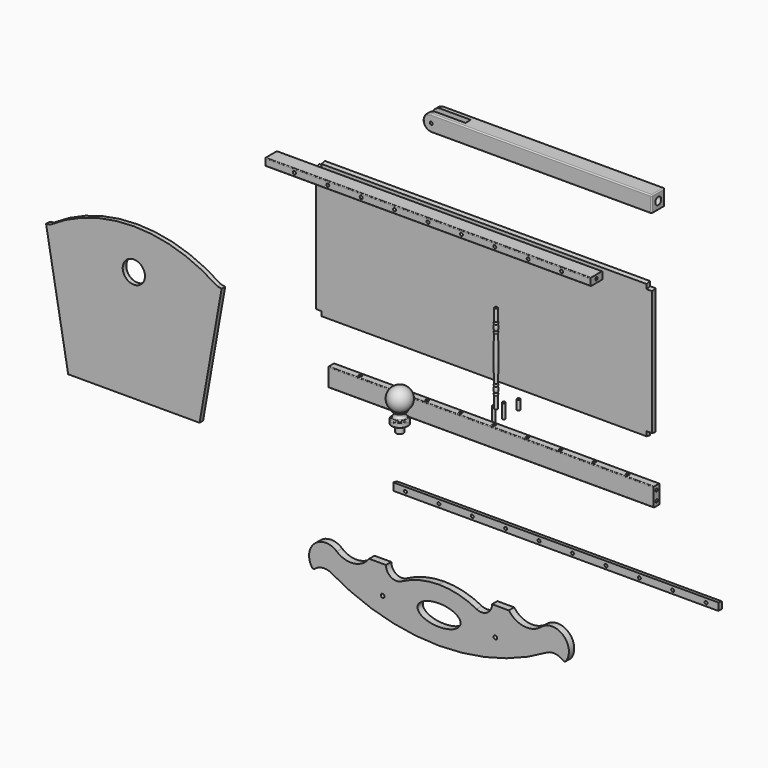
from build123d import *

# Parameters (mm, degrees)
F0_W      = 876
F0_H      = 20
F1_DEPTH  = 50
F2_R      = 4
F4_DEPTH  = 20
F5_R      = 4
F6_DEPTH  = 20
F12_DEPTH = 18
F13_R     = 5
F14_R     = 5
F15_DEPTH = 18
F16_R     = 30
F17_DEPTH = 12
F18_W     = 876
F18_H     = 20
F19_DEPTH = 40
F20_R     = 4
F21_DEPTH = 20
F22_R     = 4
F23_DEPTH = 20
F24_R     = 4
F25_DEPTH = 20
F26_R     = 2
F27_R     = 2
F28_R     = 4
F29_DEPTH = 16
F30_R     = 2
F31_R     = 4
F32_DEPTH = 39
F33_SIZE  = 0.5
F34_R     = 4
F35_DEPTH = 44
F37_DEPTH = 44
F40_DEPTH = 18
F41_R     = 4
F42_DEPTH = 180.001
F43_DEPTH = 20
F44_W     = 345
F44_H     = 12
F45_DEPTH = 12
F46_R     = 10
F47_DEPTH = 20
F48_R     = 3
F50_DEPTH = 876
F51_R     = 4
F52_DEPTH = 12
F53_R     = 4
F54_DEPTH = 27
F55_SIZE  = 1
F57_DEPTH = 906
F59_DEPTH = 15
F61_DEPTH = 15


# Not quite as in the source:
# - a pattern or mirror of a feature is missing from the dataset's text; its kind, count and spacing are read off the source's solid


with BuildPart() as f1:
    # F0 (on Top) → F1 (new body)
    with BuildSketch(Plane.XY):
        with Locations((62, 90)):
            Rectangle(F0_W, F0_H)
    extrude(amount=F1_DEPTH)

    # F2 (on face) → F4 (cut)
    with BuildSketch(Plane(origin=(-376, 0, 0), x_dir=(0, -1, 0), z_dir=(-1, 0, 0))):
        with Locations((-90, 38)):
            Circle(F2_R)
        with Locations((-90, 12)):
            Circle(F2_R)
    f4 = extrude(amount=-F4_DEPTH, mode=Mode.SUBTRACT)

    # F4_copies: F4 across plane
    add(f4.mirror(Plane(origin=(62, 0, 0), x_dir=(0, 0, 1), z_dir=(1, 0, 0))), mode=Mode.SUBTRACT)

    # F5 (on face) → F6 (cut)
    with BuildSketch(Plane.XY.offset(50)):
        with Locations((-298, 90)):
            Circle(F5_R)
        with Locations((-208, 90)):
            Circle(F5_R)
        with Locations((-118, 90)):
            Circle(F5_R)
        with Locations((-28, 90)):
            Circle(F5_R)
        with Locations((62, 90)):
            Circle(F5_R)
        with Locations((152, 90)):
            Circle(F5_R)
        with Locations((242, 90)):
            Circle(F5_R)
        with Locations((332, 90)):
            Circle(F5_R)
        with Locations((422, 90)):
            Circle(F5_R)
    extrude(amount=-F6_DEPTH, mode=Mode.SUBTRACT)

    # F27
    f27_edges = [f1.edges().sort_by_distance(p)[0] for p in [
        (62, 80, 50),
        (62, 100, 50),
        (62, 80, 0),
        (62, 100, 0),
    ]]
    fillet(f27_edges, radius=F27_R)

    # F28 (on face) → F29 (cut)
    with BuildSketch(Plane(origin=(0, 100, 0), x_dir=(-1, 0, 0), z_dir=(0, 1, 0))):
        with Locations((-467, 12)):
            Circle(F28_R)
        with Locations((-377, 12)):
            Circle(F28_R)
        with Locations((-287, 12)):
            Circle(F28_R)
        with Locations((-197, 12)):
            Circle(F28_R)
        with Locations((-107, 12)):
            Circle(F28_R)
        with Locations((-17, 12)):
            Circle(F28_R)
        with Locations((73, 12)):
            Circle(F28_R)
        with Locations((163, 12)):
            Circle(F28_R)
        with Locations((253, 12)):
            Circle(F28_R)
        with Locations((343, 12)):
            Circle(F28_R)
    extrude(amount=-F29_DEPTH, mode=Mode.SUBTRACT)


with BuildPart() as f8:
    # F7 (on Front) → F8 (revolve)
    with BuildSketch(Plane.XZ):
        with BuildLine():
            Line((139.2944970131, 150), (139.2944970131, 390))
            Line((139.2944970131, 390), (135.2944970131, 390))
            Line((135.2944970131, 390), (135.2944970131, 370))
            Line((135.2944970131, 370), (135.2944970131, 358))
            ThreePointArc((135.2944970131, 358), (134.2717225881, 354.5), (135.2944970131, 351))
            ThreePointArc((135.2944970131, 351), (133.8349932308, 343.5), (135.2944970131, 336))
            ThreePointArc((135.2944970131, 336), (134.2717225881, 332.5), (135.2944970131, 329))
            ThreePointArc((135.2944970131, 329), (133.8432027401, 270), (135.2944970131, 211))
            ThreePointArc((135.2944970131, 211), (134.2717225881, 207.5), (135.2944970131, 204))
            ThreePointArc((135.2944970131, 204), (133.8349932308, 196.5), (135.2944970131, 189))
            ThreePointArc((135.2944970131, 189), (134.2717225881, 185.5), (135.2944970131, 182))
            Line((135.2944970131, 182), (135.2944970131, 170))
            Line((135.2944970131, 170), (135.2944970131, 150))
            Line((135.2944970131, 150), (139.2944970131, 150))
        make_face()
    revolve(axis=Axis((139.2944970131, 0, 270), (0, 0, -1)))


with BuildPart() as f10:
    # F9 (on Right) → F10 (revolve)
    with BuildSketch(Plane.YZ):
        with BuildLine():
            Line((-150, 110.7184141886), (-150, 220))
            ThreePointArc((-150, 220), (-178.6491921846, 198.9007745265), (-167, 165.2815858114))
            Line((-167, 165.2815858114), (-167, 160.2815858114))
            ThreePointArc((-167, 160.2815858114), (-160.7184141886, 154), (-167, 147.7184141886))
            Line((-167, 147.7184141886), (-167, 142.7184141886))
            Line((-167, 142.7184141886), (-172, 142.7184141886))
            Line((-172, 142.7184141886), (-172, 130.7184141886))
            Line((-172, 130.7184141886), (-160, 130.7184141886))
            Line((-160, 130.7184141886), (-160, 110.7184141886))
            Line((-160, 110.7184141886), (-150, 110.7184141886))
        make_face()
    revolve(axis=Axis((0, -150, 165.3592070943), (0, 0, -1)))

    # F30
    f30_edges = [f10.edges().sort_by_distance(p)[0] for p in [
        (0, -133, 165.281586),
        (0, -133, 160.281586),
        (0, -133, 147.718414),
        (0, -133, 142.718414),
        (0, -128, 142.718414),
        (0, -128, 130.718414),
    ]]
    fillet(f30_edges, radius=F30_R)


with BuildPart() as f12:
    # F11 (on Front) → F12 (new body)
    with BuildSketch(Plane.XZ):
        with BuildLine():
            ThreePointArc((-188.266028276, -305), (-229.4682135143, -329.5253911565), (-275.4805216361, -316.0353066093))
            ThreePointArc((-275.4805216361, -316.0353066093), (-337.0528643075, -318.4149736475), (-338.527017166, -380.0156479182))
            ThreePointArc((-338.527017166, -380.0156479182), (-317.9715095123, -368.0190813721), (-294.2398267354, -369.8228929958))
            ThreePointArc((-294.2398267354, -369.8228929958), (-152.4839697516, -429.5968539661), (0, -450))
            ThreePointArc((0, -450), (152.4839697516, -429.5968539661), (294.2398267354, -369.8228929958))
            ThreePointArc((294.2398267354, -369.8228929958), (317.9715095123, -368.0190813721), (338.527017166, -380.0156479182))
            ThreePointArc((338.527017166, -380.0156479182), (337.0528643075, -318.4149736475), (275.4805216361, -316.0353066093))
            ThreePointArc((275.4805216361, -316.0353066093), (229.4682135143, -329.5253911565), (188.266028276, -305))
            Line((188.266028276, -305), (143, -305))
            ThreePointArc((143, -305), (129.1882379716, -329.4234654644), (101.139953313, -330.1745735321))
            ThreePointArc((101.139953313, -330.1745735321), (52.1129765718, -311.388216931), (0, -305))
            ThreePointArc((0, -305), (-52.1129765718, -311.388216931), (-101.139953313, -330.1745735321))
            ThreePointArc((-101.139953313, -330.1745735321), (-129.1882379716, -329.4234654644), (-143, -305))
            Line((-143, -305), (-188.266028276, -305))
        make_face()
    extrude(amount=F12_DEPTH)

    # F13
    f13_edges = [f12.edges().sort_by_distance(p)[0] for p in [
        (-338.527017, -9, -380.015648),
        (338.527017, -9, -380.015648),
    ]]
    fillet(f13_edges, radius=F13_R)

    # F14 (on face) → F15 (cut, through all)
    with BuildSketch(Plane.XZ.offset(18)):
        with Locations((-151.8835, -381)):
            Circle(F14_R)
        with BuildLine():
            add(Edge.make_bspline(
                [(58, -377.5), (58, -329.0025773881), (-29, -353.251288694), (-116, -377.5), (-29, -401.748711306), (58, -425.9974226119), (58, -377.5)],
                knots=[0, 0, 0, 2.0943951024, 2.0943951024, 4.1887902048, 4.1887902048, 6.2831853072, 6.2831853072, 6.2831853072], degree=2, weights=[1, 0.5, 1, 0.5, 1, 0.5, 1]))
        make_face()
        with Locations((151.8835, -381)):
            Circle(F14_R)
    extrude(amount=-F15_DEPTH, mode=Mode.SUBTRACT)


with BuildPart() as f17:
    # F16 (on Front) → F17 (new body)
    with BuildSketch(Plane.XZ):
        with BuildLine():
            Line((-1004, -135), (-650, -135))
            Line((-650, -135), (-590.5, 202.4412682673))
            Line((-590.5, 202.4412682673), (-602.3176930361, 204.5250463993))
            ThreePointArc((-602.3176930361, 204.5250463993), (-827, 273.5902175622), (-1051.6823069639, 204.5250463993))
            Line((-1051.6823069639, 204.5250463993), (-1063.5, 202.4412682673))
            Line((-1063.5, 202.4412682673), (-1004, -135))
        make_face()
        with Locations((-827, 165)):
            Circle(F16_R, mode=Mode.SUBTRACT)
    extrude(amount=F17_DEPTH)


with BuildPart() as f19:
    # F18 (on Front) → F19 (new body)
    with BuildSketch(Plane.XZ):
        with Locations((-12, 560)):
            Rectangle(F18_W, F18_H)
    extrude(amount=F19_DEPTH)

    # F20 (on face) → F21 (cut)
    with BuildSketch(Plane.XZ.offset(40)):
        with Locations((-372, 560)):
            Circle(F20_R)
        with Locations((-282, 560)):
            Circle(F20_R)
        with Locations((-192, 560)):
            Circle(F20_R)
        with Locations((-102, 560)):
            Circle(F20_R)
        with Locations((-12, 560)):
            Circle(F20_R)
        with Locations((78, 560)):
            Circle(F20_R)
        with Locations((168, 560)):
            Circle(F20_R)
        with Locations((348, 560)):
            Circle(F20_R)
        with Locations((258, 560)):
            Circle(F20_R)
    extrude(amount=-F21_DEPTH, mode=Mode.SUBTRACT)

    # F22 (on face) → F23 (cut)
    with BuildSketch(Plane.YZ.offset(426)):
        with Locations((-20, 560)):
            Circle(F22_R)
    extrude(amount=-F23_DEPTH, mode=Mode.SUBTRACT)

    # F24 (on face) → F25 (cut)
    with BuildSketch(Plane(origin=(-450, 0, 0), x_dir=(0, -1, 0), z_dir=(-1, 0, 0))):
        with Locations((20, 560)):
            Circle(F24_R)
    extrude(amount=-F25_DEPTH, mode=Mode.SUBTRACT)

    # F26
    f26_edges = [f19.edges().sort_by_distance(p)[0] for p in [
        (-12, -40, 550),
        (-12, 0, 550),
        (-12, -40, 570),
        (-12, 0, 570),
    ]]
    fillet(f26_edges, radius=F26_R)


with BuildPart() as f32:
    # F31 (on Top) → F32 (new body)
    with BuildSketch(Plane.XY):
        with Locations((0, 200)):
            Circle(F31_R)
    extrude(amount=F32_DEPTH)

    # F33
    f33_edges = [f32.edges().sort_by_distance(p)[0] for p in [
        (-4, 200, 39),
        (-4, 200, 0),
    ]]
    chamfer(f33_edges, length=F33_SIZE)


with BuildPart() as f35:
    # F34 (on Top) → F35 (new body)
    with BuildSketch(Plane.XY):
        with Locations((0, 166.5)):
            Circle(F34_R)
    extrude(amount=F35_DEPTH)


with BuildPart() as f37:
    # F36 (on Front) → F37 (new body)
    with BuildSketch(Plane.XZ):
        with BuildLine():
            Line((594, 822), (0, 822))
            ThreePointArc((0, 822), (-22, 800), (0, 778))
            Line((0, 778), (594, 778))
            Line((594, 778), (594, 822))
        make_face()
    extrude(amount=F37_DEPTH)

    # F39 (on offset) → F40 (cut)
    with BuildSketch(Plane(origin=(0, -13, 0), x_dir=(-1, 0, 0), z_dir=(0, 1, 0))):
        Polygon((-74, 778), (22, 778), (22, 822), (-81.7583871512, 822), align=None)
    extrude(amount=-F40_DEPTH, mode=Mode.SUBTRACT)

    # F41 (on face) → F42 (cut, through all)
    with BuildSketch(Plane(origin=(0, 0, 0), x_dir=(-1, 0, 0), z_dir=(0, 1, 0))):
        with Locations((0, 800)):
            Circle(F41_R)
    extrude(amount=-F42_DEPTH, mode=Mode.SUBTRACT)

    # F41 (on face) → F43 (cut)
    with BuildSketch(Plane(origin=(0, 0, 0), x_dir=(-1, 0, 0), z_dir=(0, 1, 0))):
        with Locations((-218, 800)):
            Circle(F41_R)
        with Locations((-244, 800)):
            Circle(F41_R)
        with Locations((-481, 800)):
            Circle(F41_R)
    extrude(amount=-F43_DEPTH, mode=Mode.SUBTRACT)

    # F44 (on face) → F45 (cut)
    with BuildSketch(Plane(origin=(0, 0, 778), x_dir=(1, 0, 0), z_dir=(0, 0, -1))):
        with Locations((371.5, 22)):
            Rectangle(F44_W, F44_H)
    extrude(amount=-F45_DEPTH, mode=Mode.SUBTRACT)

    # F46 (on face) → F47 (cut)
    with BuildSketch(Plane.YZ.offset(594)):
        with Locations((-22, 800)):
            Circle(F46_R)
    extrude(amount=-F47_DEPTH, mode=Mode.SUBTRACT)

    # F48
    f48_edges = [f37.edges().sort_by_distance(p)[0] for p in [
        (297, -44, 822),
        (297, 0, 822),
        (594, 0, 800),
        (594, -22, 822),
        (594, -44, 800),
        (594, -22, 778),
        (297, 0, 778),
        (297, -44, 778),
        (-22, 0, 800),
        (-22, -44, 800),
    ]]
    fillet(f48_edges, radius=F48_R)


with BuildPart() as f50:
    # F49 (on Right) → F50 (new body)
    with BuildSketch(Plane.YZ):
        Polygon((-160, -2.1159237685), (-172, 0), (-172, -20), (-160, -20), align=None)
    extrude(amount=F50_DEPTH)

    # F51 (on face) → F52 (cut, through all)
    with BuildSketch(Plane.XZ.offset(172)):
        with Locations((33, -11)):
            Circle(F51_R)
        with Locations((123, -11)):
            Circle(F51_R)
        with Locations((213, -11)):
            Circle(F51_R)
        with Locations((303, -11)):
            Circle(F51_R)
        with Locations((393, -11)):
            Circle(F51_R)
        with Locations((483, -11)):
            Circle(F51_R)
        with Locations((573, -11)):
            Circle(F51_R)
        with Locations((663, -11)):
            Circle(F51_R)
        with Locations((753, -11)):
            Circle(F51_R)
        with Locations((843, -11)):
            Circle(F51_R)
    extrude(amount=-F52_DEPTH, mode=Mode.SUBTRACT)


with BuildPart() as f54:
    # F53 (on Top) → F54 (new body)
    with BuildSketch(Plane.XY):
        with Locations((0, 250)):
            Circle(F53_R)
    extrude(amount=F54_DEPTH)

    # F55
    f55_edges = [f54.edges().sort_by_distance(p)[0] for p in [
        (-4, 250, 27),
        (-4, 250, 0),
    ]]
    chamfer(f55_edges, length=F55_SIZE)


with BuildPart() as f57:
    # F56 (on Right) → F57 (new body)
    with BuildSketch(Plane.YZ):
        Polygon((712, -252.1159237685), (712, 113.3840762315), (700, 111.268152463), (700, -250), align=None)
    extrude(amount=-F57_DEPTH)

    # F58 (on face) → F59 (cut)
    with BuildSketch(Plane(origin=(-906, 0, 0), x_dir=(0, -1, 0), z_dir=(-1, 0, 0))):
        Polygon((-700, 111.268152463), (-712, 113.3840762315), (-712, 101.1989568889), (-700, 99.0830331204), align=None)
        Polygon((-700, -237.8148806574), (-712, -239.9308044259), (-712, -252.1159237685), (-700, -250), align=None)
    extrude(amount=-F59_DEPTH, mode=Mode.SUBTRACT)

    # F60 (on face) → F61 (cut)
    with BuildSketch(Plane.YZ):
        Polygon((712, 113.3840762315), (700, 111.268152463), (700, 99.0830331204), (712, 101.1989568889), align=None)
        Polygon((712, -239.9308044259), (700, -237.8148806574), (700, -250), (712, -252.1159237685), align=None)
    extrude(amount=-F61_DEPTH, mode=Mode.SUBTRACT)


solid = Compound([f1.part, f8.part, f10.part, f12.part, f17.part, f19.part, f32.part, f35.part, f37.part, f50.part, f54.part, f57.part])
